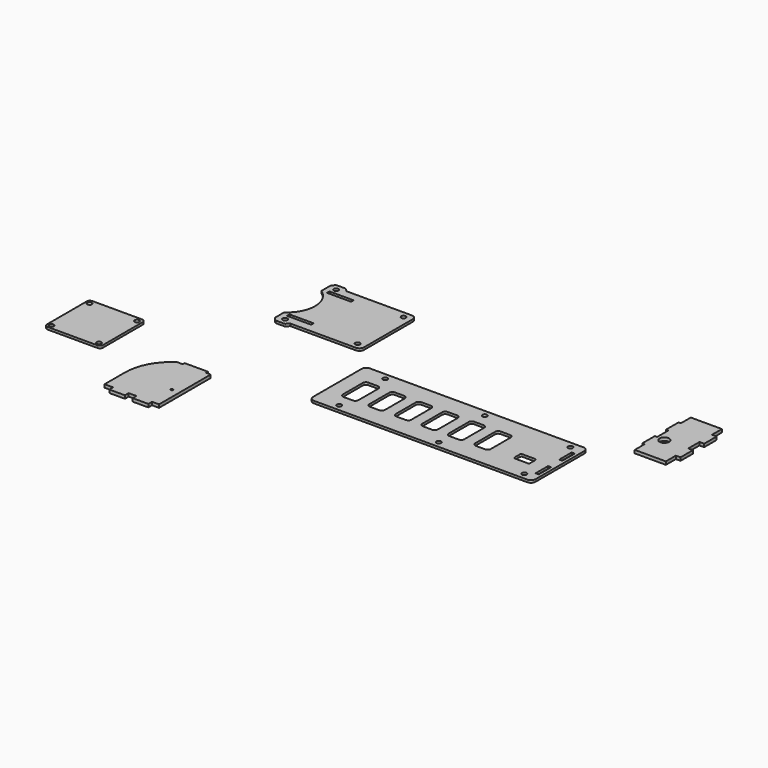
from build123d import *

# Parameters (mm, degrees)
F0_R     = 1.5
F0_W     = 15.5
F0_H     = 2
F1_DEPTH = 1.5
F0_W_2   = 2
F0_H_2   = 10
F0_R_2   = 3.05
F0_W_3   = 3
F0_W_4   = 1.5
F0_R_3   = 0.75
F0_W_5   = 15
F0_H_3   = 1.5
F0_W_6   = 10
F0_H_4   = 3
F2_DEPTH = 0.5


# Not quite as in the source:
# - a feature names something its author has since deleted; it is built from what else it names


with BuildPart() as f1:
    # F0 (on Top) → F1 (new body)
    with BuildSketch(Plane.XY):
        with BuildLine():
            Line((14.7071067812, 96.1655887486), (13, 94.4584819674))
            Line((13, 94.4584819674), (13, 86.9584819674))
            ThreePointArc((13, 86.9584819674), (20.8733394058, 71.9584819674), (13, 56.9584819674))
            Line((13, 56.9584819674), (13, 49.4584819674))
            Line((13, 49.4584819674), (14.7071067812, 47.7513751863))
            ThreePointArc((14.7071067812, 47.7513751863), (15.03153013, 47.5346024349), (15.4142135624, 47.4584819674))
            Line((15.4142135624, 47.4584819674), (20.5857864376, 47.4584819674))
            ThreePointArc((20.5857864376, 47.4584819674), (20.96846987, 47.5346024349), (21.2928932188, 47.7513751863))
            Line((21.2928932188, 47.7513751863), (23, 49.4584819674))
            Line((23, 49.4584819674), (65, 49.4584819674))
            ThreePointArc((65, 49.4584819674), (67.1213203436, 50.3371616239), (68, 52.4584819674))
            Line((68, 52.4584819674), (68, 91.4584819674))
            ThreePointArc((68, 91.4584819674), (67.1213203436, 93.579802311), (65, 94.4584819674))
            Line((65, 94.4584819674), (23, 94.4584819674))
            Line((23, 94.4584819674), (21.2928932188, 96.1655887486))
            ThreePointArc((21.2928932188, 96.1655887486), (20.96846987, 96.3823615), (20.5857864376, 96.4584819674))
            Line((20.5857864376, 96.4584819674), (15.4142135624, 96.4584819674))
            ThreePointArc((15.4142135624, 96.4584819674), (15.03153013, 96.3823615), (14.7071067812, 96.1655887486))
        make_face()
        with Locations((18, 51.4584819674)):
            Circle(F0_R, mode=Mode.SUBTRACT)
        with Locations((24.25, 55.9584819674)):
            Rectangle(F0_W, F0_H, mode=Mode.SUBTRACT)
        with Locations((63, 53.4584819674)):
            Circle(F0_R, mode=Mode.SUBTRACT)
        with Locations((24.25, 87.9584819674)):
            Rectangle(F0_W, F0_H, mode=Mode.SUBTRACT)
        with Locations((18, 92.4584819674)):
            Circle(F0_R, mode=Mode.SUBTRACT)
        with Locations((63, 90.4584819674)):
            Circle(F0_R, mode=Mode.SUBTRACT)
    extrude(amount=F1_DEPTH)


with BuildPart() as f1b:
    # F0 (on Top) → F1, piece 2 (new body)
    with BuildSketch(Plane.XY):
        with BuildLine():
            Line((-37.7851966619, 6.4972268343), (-69.7851966619, 6.4972268343))
            ThreePointArc((-69.7851966619, 6.4972268343), (-71.1994102243, 5.9114403967), (-71.7851966619, 4.4972268343))
            Line((-71.7851966619, 4.4972268343), (-71.7851966619, -27.5027731657))
            ThreePointArc((-71.7851966619, -27.5027731657), (-71.1994102243, -28.9169867281), (-69.7851966619, -29.5027731657))
            Line((-69.7851966619, -29.5027731657), (-37.7851966619, -29.5027731657))
            ThreePointArc((-37.7851966619, -29.5027731657), (-36.3709830996, -28.9169867281), (-35.7851966619, -27.5027731657))
            Line((-35.7851966619, -27.5027731657), (-35.7851966619, 4.4972268343))
            ThreePointArc((-35.7851966619, 4.4972268343), (-36.3709830996, 5.9114403967), (-37.7851966619, 6.4972268343))
        make_face()
        with Locations((-69.2351966619, -26.9527731657)):
            Circle(F0_R, mode=Mode.SUBTRACT)
        with Locations((-38.7351966619, -26.9527731657)):
            Circle(F0_R, mode=Mode.SUBTRACT)
        with Locations((-69.2351966619, 3.5472268343)):
            Circle(F0_R, mode=Mode.SUBTRACT)
        with Locations((-38.7351966619, 3.5472268343)):
            Circle(F0_R, mode=Mode.SUBTRACT)
    extrude(amount=F1_DEPTH)


with BuildPart() as f1c:
    # F0 (on Top) → F1, piece 3 (new body)
    with BuildSketch(Plane.XY):
        with BuildLine():
            Line((224.6754089409, -5.6948737871), (224.6754089409, 33.3051262129))
            ThreePointArc((224.6754089409, 33.3051262129), (223.7967292845, 35.4264465564), (221.6754089409, 36.3051262129))
            Line((221.6754089409, 36.3051262129), (84.6754089409, 36.3051262129))
            ThreePointArc((84.6754089409, 36.3051262129), (82.5540885974, 35.4264465564), (81.6754089409, 33.3051262129))
            Line((81.6754089409, 33.3051262129), (81.6754089409, -5.6948737871))
            ThreePointArc((81.6754089409, -5.6948737871), (82.5540885974, -7.8161941307), (84.6754089409, -8.6948737871))
            Line((84.6754089409, -8.6948737871), (221.6754089409, -8.6948737871))
            ThreePointArc((221.6754089409, -8.6948737871), (223.7967292845, -7.8161941307), (224.6754089409, -5.6948737871))
        make_face()
        with Locations((97.6754089409, -4.6948737871)):
            Circle(F0_R, mode=Mode.SUBTRACT)
        with BuildLine():
            ThreePointArc((91.6754089409, 21.8051262129), (92.2611953786, 23.2193397752), (93.6754089409, 23.8051262129))
            Line((93.6754089409, 23.8051262129), (99.6754089409, 23.8051262129))
            ThreePointArc((99.6754089409, 23.8051262129), (101.0896225033, 23.2193397752), (101.6754089409, 21.8051262129))
            Line((101.6754089409, 21.8051262129), (101.6754089409, 5.8051262129))
            ThreePointArc((101.6754089409, 5.8051262129), (101.0896225033, 4.3909126505), (99.6754089409, 3.8051262129))
            Line((99.6754089409, 3.8051262129), (93.6754089409, 3.8051262129))
            ThreePointArc((93.6754089409, 3.8051262129), (92.2611953786, 4.3909126505), (91.6754089409, 5.8051262129))
            Line((91.6754089409, 5.8051262129), (91.6754089409, 21.8051262129))
        make_face(mode=Mode.SUBTRACT)
        with Locations((161.6754089409, -4.6948737871)):
            Circle(F0_R, mode=Mode.SUBTRACT)
        with BuildLine():
            ThreePointArc((108.6754089409, 21.8051262129), (109.2611953786, 23.2193397752), (110.6754089409, 23.8051262129))
            Line((110.6754089409, 23.8051262129), (116.6754089409, 23.8051262129))
            ThreePointArc((116.6754089409, 23.8051262129), (118.0896225033, 23.2193397752), (118.6754089409, 21.8051262129))
            Line((118.6754089409, 21.8051262129), (118.6754089409, 5.8051262129))
            ThreePointArc((118.6754089409, 5.8051262129), (118.0896225033, 4.3909126505), (116.6754089409, 3.8051262129))
            Line((116.6754089409, 3.8051262129), (110.6754089409, 3.8051262129))
            ThreePointArc((110.6754089409, 3.8051262129), (109.2611953786, 4.3909126505), (108.6754089409, 5.8051262129))
            Line((108.6754089409, 5.8051262129), (108.6754089409, 21.8051262129))
        make_face(mode=Mode.SUBTRACT)
        with BuildLine():
            ThreePointArc((125.6754089409, 21.8051262129), (126.2611953786, 23.2193397752), (127.6754089409, 23.8051262129))
            Line((127.6754089409, 23.8051262129), (133.6754089409, 23.8051262129))
            ThreePointArc((133.6754089409, 23.8051262129), (135.0896225033, 23.2193397752), (135.6754089409, 21.8051262129))
            Line((135.6754089409, 21.8051262129), (135.6754089409, 5.8051262129))
            ThreePointArc((135.6754089409, 5.8051262129), (135.0896225033, 4.3909126505), (133.6754089409, 3.8051262129))
            Line((133.6754089409, 3.8051262129), (127.6754089409, 3.8051262129))
            ThreePointArc((127.6754089409, 3.8051262129), (126.2611953786, 4.3909126505), (125.6754089409, 5.8051262129))
            Line((125.6754089409, 5.8051262129), (125.6754089409, 21.8051262129))
        make_face(mode=Mode.SUBTRACT)
        with BuildLine():
            ThreePointArc((142.6754089409, 21.8051262129), (143.2611953786, 23.2193397752), (144.6754089409, 23.8051262129))
            Line((144.6754089409, 23.8051262129), (150.6754089409, 23.8051262129))
            ThreePointArc((150.6754089409, 23.8051262129), (152.0896225033, 23.2193397752), (152.6754089409, 21.8051262129))
            Line((152.6754089409, 21.8051262129), (152.6754089409, 5.8051262129))
            ThreePointArc((152.6754089409, 5.8051262129), (152.0896225033, 4.3909126505), (150.6754089409, 3.8051262129))
            Line((150.6754089409, 3.8051262129), (144.6754089409, 3.8051262129))
            ThreePointArc((144.6754089409, 3.8051262129), (143.2611953786, 4.3909126505), (142.6754089409, 5.8051262129))
            Line((142.6754089409, 5.8051262129), (142.6754089409, 21.8051262129))
        make_face(mode=Mode.SUBTRACT)
        with BuildLine():
            ThreePointArc((159.6754089409, 21.8051262129), (160.2611953786, 23.2193397752), (161.6754089409, 23.8051262129))
            Line((161.6754089409, 23.8051262129), (167.6754089409, 23.8051262129))
            ThreePointArc((167.6754089409, 23.8051262129), (169.0896225033, 23.2193397752), (169.6754089409, 21.8051262129))
            Line((169.6754089409, 21.8051262129), (169.6754089409, 5.8051262129))
            ThreePointArc((169.6754089409, 5.8051262129), (169.0896225033, 4.3909126505), (167.6754089409, 3.8051262129))
            Line((167.6754089409, 3.8051262129), (161.6754089409, 3.8051262129))
            ThreePointArc((161.6754089409, 3.8051262129), (160.2611953786, 4.3909126505), (159.6754089409, 5.8051262129))
            Line((159.6754089409, 5.8051262129), (159.6754089409, 21.8051262129))
        make_face(mode=Mode.SUBTRACT)
        with BuildLine():
            ThreePointArc((176.6754089409, 21.8051262129), (177.2611953786, 23.2193397752), (178.6754089409, 23.8051262129))
            Line((178.6754089409, 23.8051262129), (184.6754089409, 23.8051262129))
            ThreePointArc((184.6754089409, 23.8051262129), (186.0896225033, 23.2193397752), (186.6754089409, 21.8051262129))
            Line((186.6754089409, 21.8051262129), (186.6754089409, 5.8051262129))
            ThreePointArc((186.6754089409, 5.8051262129), (186.0896225033, 4.3909126505), (184.6754089409, 3.8051262129))
            Line((184.6754089409, 3.8051262129), (178.6754089409, 3.8051262129))
            ThreePointArc((178.6754089409, 3.8051262129), (177.2611953786, 4.3909126505), (176.6754089409, 5.8051262129))
            Line((176.6754089409, 5.8051262129), (176.6754089409, 21.8051262129))
        make_face(mode=Mode.SUBTRACT)
        with Locations((216.6754089409, -4.6948737871)):
            Circle(F0_R, mode=Mode.SUBTRACT)
        with Locations((221.6754089409, 4.3051262129)):
            Rectangle(F0_W_2, F0_H_2, mode=Mode.SUBTRACT)
        with BuildLine():
            Line((211.6754089409, 10.3051262129), (211.6754089409, 6.3051262129))
            ThreePointArc((211.6754089409, 6.3051262129), (211.3825157221, 5.5980194317), (210.6754089409, 5.3051262129))
            Line((210.6754089409, 5.3051262129), (202.6754089409, 5.3051262129))
            ThreePointArc((202.6754089409, 5.3051262129), (201.9683021597, 5.5980194317), (201.6754089409, 6.3051262129))
            Line((201.6754089409, 6.3051262129), (201.6754089409, 10.3051262129))
            ThreePointArc((201.6754089409, 10.3051262129), (201.9683021597, 11.0122329941), (202.6754089409, 11.3051262129))
            Line((202.6754089409, 11.3051262129), (210.6754089409, 11.3051262129))
            ThreePointArc((210.6754089409, 11.3051262129), (211.3825157221, 11.0122329941), (211.6754089409, 10.3051262129))
        make_face(mode=Mode.SUBTRACT)
        with Locations((97.6754089409, 32.3051262129)):
            Circle(F0_R, mode=Mode.SUBTRACT)
        with Locations((161.6754089409, 32.3051262129)):
            Circle(F0_R, mode=Mode.SUBTRACT)
        with Locations((221.6754089409, 23.3051262129)):
            Rectangle(F0_W_2, F0_H_2, mode=Mode.SUBTRACT)
        with Locations((216.6754089409, 32.3051262129)):
            Circle(F0_R, mode=Mode.SUBTRACT)
    extrude(amount=F1_DEPTH)


with BuildPart() as f1d:
    # F0 (on Top) → F1, piece 4 (new body)
    with BuildSketch(Plane.XY):
        Polygon((264.2433282137, 94.4584819674), (244.2433282137, 94.4584819674), (244.2433282137, 86.4584819674), (244.2433282137, 76.4584819674), (244.2433282137, 67.4584819674), (244.2433282137, 57.4584819674), (244.2433282137, 49.4584819674), (264.2433282137, 49.4584819674), (264.2433282137, 57.4584819674), (264.2433282137, 67.4584819674), (264.2433282137, 76.4584819674), (264.2433282137, 86.4584819674), align=None)
        with Locations((249.2433282137, 66.9584819674)):
            Circle(F0_R_2, mode=Mode.SUBTRACT)
        with Locations((265.7433282137, 81.4584819674)):
            Rectangle(F0_W_3, F0_H_2)
        with Locations((265.7433282137, 62.4584819674)):
            Rectangle(F0_W_3, F0_H_2)
        with Locations((243.4933282137, 62.4584819674)):
            Rectangle(F0_W_4, F0_H_2)
        with Locations((243.4933282137, 81.4584819674)):
            Rectangle(F0_W_4, F0_H_2)
    extrude(amount=F1_DEPTH)

    # F2#2 (add): a face of the model
    f2_2_faces = [f1d.faces().sort_by_distance(p)[0] for p in [
        (254.7779207557, 72.1105709346, 1.5),
    ]]
    extrude(f2_2_faces, amount=F2_DEPTH)


with BuildPart() as f1e:
    # F0 (on Top) → F1, piece 5 (new body)
    with BuildSketch(Plane.XY):
        with BuildLine():
            Line((-7.9848988752, -44.4907953074), (-7.9848988752, -60.9907953074))
            Line((-7.9848988752, -60.9907953074), (-2.4848988752, -60.9907953074))
            Line((-2.4848988752, -60.9907953074), (7.5151011248, -60.9907953074))
            Line((7.5151011248, -60.9907953074), (12.5151011248, -60.9907953074))
            Line((12.5151011248, -60.9907953074), (22.5151011248, -60.9907953074))
            Line((22.5151011248, -60.9907953074), (27.0151011248, -60.9907953074))
            Line((27.0151011248, -60.9907953074), (27.0151011248, -19.4907953074))
            Line((27.0151011248, -19.4907953074), (24.0151011248, -19.4907953074))
            Line((24.0151011248, -19.4907953074), (9.0151011248, -19.4907953074))
            Line((9.0151011248, -19.4907953074), (5.431977173, -19.4907953074))
            ThreePointArc((5.431977173, -19.4907953074), (-4.4187192438, -30.3044236528), (-7.9848988752, -44.4907953074))
        make_face()
        with Locations((22.0151011248, -44.4907953074)):
            Circle(F0_R_3, mode=Mode.SUBTRACT)
        with Locations((16.5151011248, -18.7407953074)):
            Rectangle(F0_W_5, F0_H_3)
        with Locations((2.5151011248, -62.4907953074)):
            Rectangle(F0_W_6, F0_H_4)
        with Locations((17.5151011248, -62.4907953074)):
            Rectangle(F0_W_6, F0_H_4)
    extrude(amount=F1_DEPTH)

    # F2 (add): a face of the model
    f2_faces = [f1e.faces().sort_by_distance(p)[0] for p in [
        (10.5800442466, -41.8563114265, 1.5),
    ]]
    extrude(f2_faces, amount=F2_DEPTH)


solid = Compound([f1.part, f1b.part, f1c.part, f1d.part, f1e.part])
